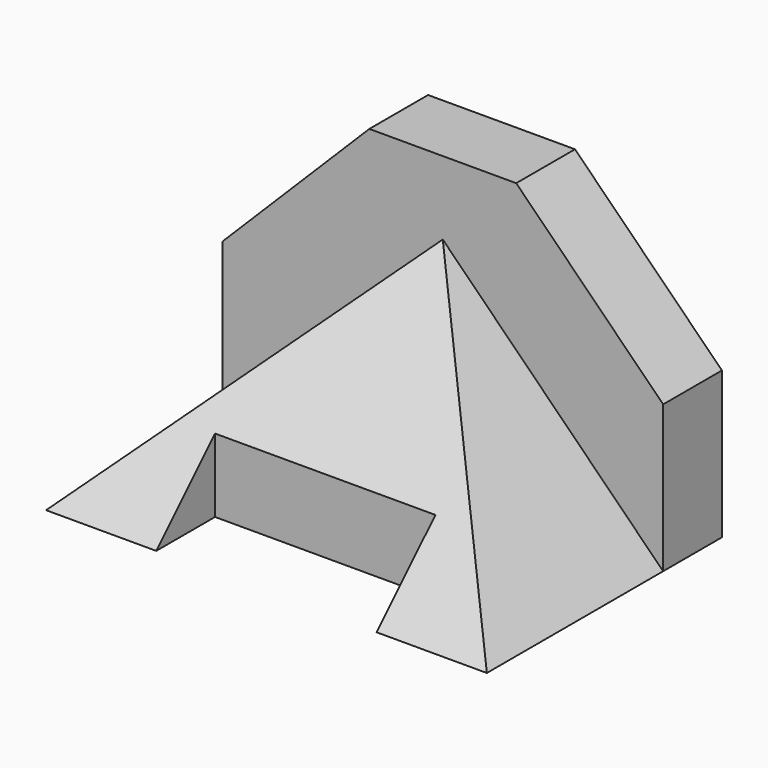
from build123d import *

# Parameters (mm, degrees)
F1_DEPTH = 12.7
F3_DEPTH = 38.1
F6_DEPTH = 35.9220244843
F8_W     = 38.1
F8_H     = 12.7
F9_DEPTH = 12.7


# Not quite as in the source:
# - a feature names something its author has since deleted; it is built from what else it names


with BuildPart() as f1:
    # F0 (on Front) → F1 (new body)
    with BuildSketch(Plane.XZ):
        Polygon((-38.1, 25.4), (-38.1, 0), (38.1, 0), (38.1, 25.4), (12.7, 50.8), (-12.7, 50.8), align=None)
    extrude(amount=F1_DEPTH)

    # F2 (on face) → F3 (join)
    with BuildSketch(Plane.XZ.offset(12.7)):
        Polygon((0, 38.1), (-38.1, 0), (38.1, 0), align=None)
    extrude(amount=F3_DEPTH)

    # F5 (on face) → F6 (cut, through all)
    with BuildSketch(Plane(origin=(0, -25.4, 25.4), x_dir=(-1, 0, 0), z_dir=(0, 0.7071067812, -0.7071067812))):
        Polygon((-38.1, -35.9210244843), (38.1, -35.9210244843), (0, 17.9605122421), align=None)
    extrude(amount=-F6_DEPTH, mode=Mode.SUBTRACT)

    # F8 (on offset) → F9 (cut)
    with BuildSketch(Plane.XZ.offset(50.8)):
        with Locations((0, 6.35)):
            Rectangle(F8_W, F8_H)
    extrude(amount=-F9_DEPTH, mode=Mode.SUBTRACT)


solid = f1.part
